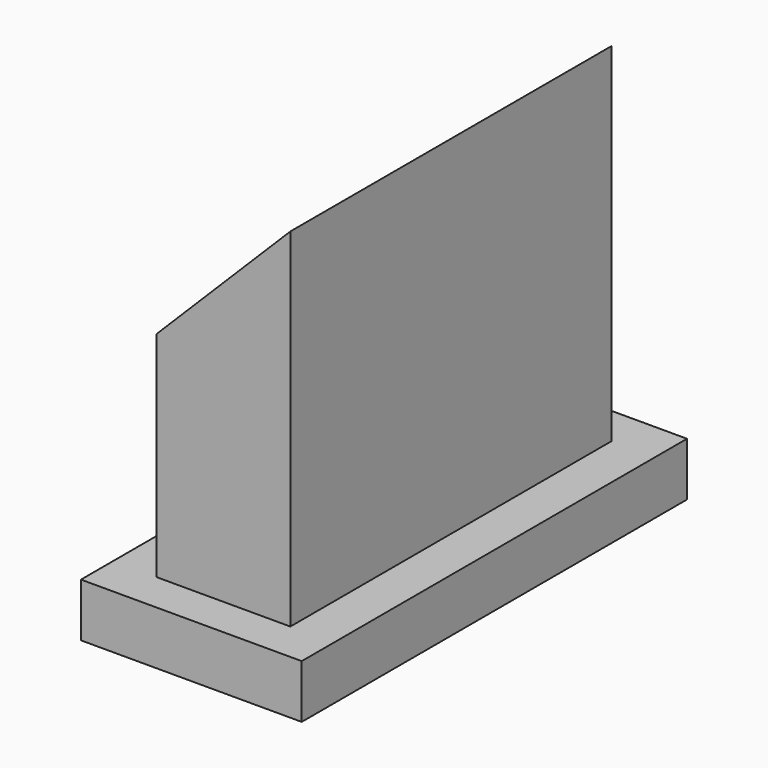
from build123d import *

# Parameters (mm, degrees)
F0_W     = 16.5
F0_H     = 36
F1_DEPTH = 4
F2_W     = 10
F2_H     = 30
F3_DEPTH = 30
F4_SIZE  = 9.99999


# Not quite as in the source:
# - a fillet or chamfer is up to 0.001 mm smaller than in the source, because OpenCascade refuses the exact size


with BuildPart() as f1:
    # F0 (on Top) → F1 (new body)
    with BuildSketch(Plane.XY):
        with Locations((8.25, 18)):
            Rectangle(F0_W, F0_H)
    extrude(amount=F1_DEPTH)

    # F2 (on Top) → F3 (join)
    with BuildSketch(Plane.XY):
        with Locations((8.25, 18)):
            Rectangle(F2_W, F2_H)
    extrude(amount=F3_DEPTH)

    # F4 (size 10 in the source; OpenCascade refuses exactly that, so slightly less here)
    f4_edges = [f1.edges().sort_by_distance(p)[0] for p in [
        (3.25, 18, 30),
    ]]
    chamfer(f4_edges, length=F4_SIZE)


solid = f1.part
